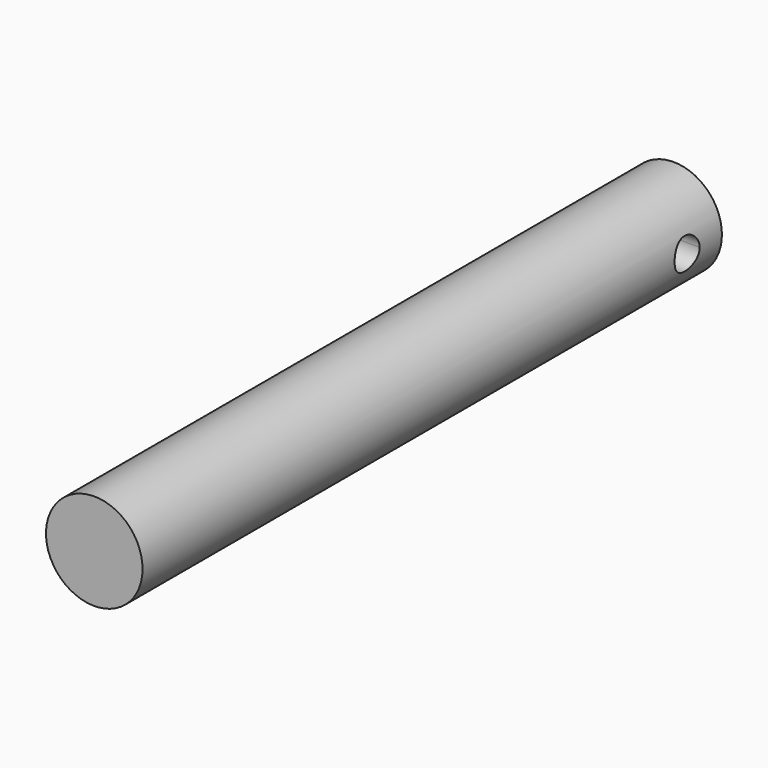
from build123d import *

# Parameters (mm, degrees)
F0_R     = 10
F1_DEPTH = 150
F4_D     = 6.5
F4_DEPTH = 10.001
F5_D     = 6.5


# Not quite as in the source:
# - a feature names something its author has since deleted; it is built from what else it names


with BuildPart() as f1:
    # F0 (on Front) → F1 (new body)
    with BuildSketch(Plane.XZ):
        Circle(F0_R)
    extrude(amount=F1_DEPTH)

    # F4 (through all, one way)
    with BuildSketch(Plane(origin=(0, 0, 0), x_dir=(0, 1, 0), z_dir=(-1, 0, 0))):
        with Locations((-9, 0)):
            Circle(F4_D / 2)
    extrude(amount=-F4_DEPTH, mode=Mode.SUBTRACT)

    # F5 (through all)
    with Locations(Plane.YZ):
        with Locations((-9, 0)):
            Hole(F5_D / 2)


solid = f1.part
